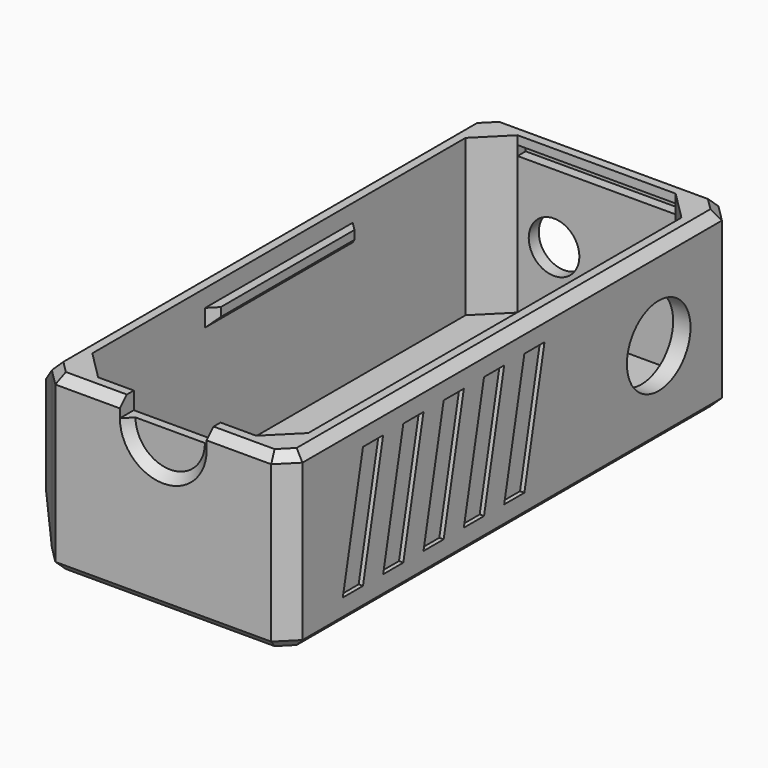
from build123d import *

# Parameters (mm, degrees)
F2_W      = 52
F2_H      = 116
F2_W_2    = 44.8
F2_H_2    = 108.8
F3_DEPTH  = 36
F4_DEPTH  = 3.6
F7_SIZE   = 3.6
F8_SIZE   = 5.9976
F6_R      = 5.25
F9_DEPTH  = 3.6
F5_R      = 8.25
F10_DEPTH = 3.6
F11_W     = 18
F11_H     = 3.6
F12_DEPTH = 3.6
F13_W     = 32.8048
F13_H     = 2
F14_DEPTH = 2.1
F6_R_2    = 12
F15_DEPTH = 1
F16_R     = 0.5
F17_W     = 38.28
F17_H     = 3.6
F19_DEPTH = 1.8
F18_W     = 38.28
F18_H     = 3.6
F20_DEPTH = 1.8
F21_SIZE  = 1.79999
F23_DEPTH = 1.8
F24_SIZE  = 1.79999
F26_W     = 89.2
F26_H     = 21.6
F27_DEPTH = 3.6
F28_DEPTH = 5.9976
F30_SIZE  = 3.59999
F29_W     = 4.775
F29_H     = 15.6718
F31_DEPTH = 2.9972
F32_SIZE  = 5.99759
F34_DEPTH = 0.9


# Not quite as in the source:
# - two fillets or chamfers of one size are made in one step
# - a fillet or chamfer is up to 0.001 mm smaller than in the source, because OpenCascade refuses the exact size


with BuildPart() as f3:
    # F2 (on Top) → F3 (new body)
    with BuildSketch(Plane.XY):
        Rectangle(F2_W, F2_H)
        Rectangle(F2_W_2, F2_H_2, mode=Mode.SUBTRACT)
    extrude(amount=F3_DEPTH)

    # F2 (on Top) → F4 (join)
    with BuildSketch(Plane.XY):
        Rectangle(F2_W_2, F2_H_2)
    extrude(amount=F4_DEPTH)

    # F7
    f7_edges = [f3.edges().sort_by_distance(p)[0] for p in [
        (-26, -58, 18),
        (26, -58, 18),
        (26, 58, 18),
        (-26, 58, 18),
    ]]
    chamfer(f7_edges, length=F7_SIZE)

    # F8
    f8_edges = [f3.edges().sort_by_distance(p)[0] for p in [
        (-22.4, 54.4, 19.8),
        (22.4, 54.4, 19.8),
        (-22.4, -54.4, 19.8),
        (22.4, -54.4, 19.8),
    ]]
    chamfer(f8_edges, length=F8_SIZE)

    # F6 (on face) → F9 (cut)
    with BuildSketch(Plane(origin=(0, 58, 0), x_dir=(-1, 0, 0), z_dir=(0, 1, 0))):
        with Locations((8.84, 18)):
            Circle(F6_R)
    extrude(amount=-F9_DEPTH, mode=Mode.SUBTRACT)

    # F5 (on face) → F10 (cut)
    with BuildSketch(Plane.YZ.offset(26)):
        with Locations((38, 18)):
            Circle(F5_R)
    extrude(amount=-F10_DEPTH, mode=Mode.SUBTRACT)

    # F11 (on face) → F12 (cut)
    with BuildSketch(Plane.XZ.offset(58)):
        with Locations((0, 34.2)):
            Rectangle(F11_W, F11_H)
    extrude(amount=-F12_DEPTH, mode=Mode.SUBTRACT)

    # F13 (on face) → F14 (cut)
    with BuildSketch(Plane.XZ.offset(-54.4)):
        with Locations((0, 33.2)):
            Rectangle(F13_W, F13_H)
    extrude(amount=-F14_DEPTH, mode=Mode.SUBTRACT)

    # F6 (on face) → F15 (cut)
    with BuildSketch(Plane(origin=(0, 58, 0), x_dir=(-1, 0, 0), z_dir=(0, 1, 0))):
        with Locations((8.84, 18)):
            Circle(F6_R_2)
        with Locations((8.84, 18)):
            Circle(F6_R, mode=Mode.SUBTRACT)
    extrude(amount=-F15_DEPTH, mode=Mode.SUBTRACT)

    # F16
    f16_edges = [f3.edges().sort_by_distance(p)[0] for p in [
        (0, 56.5, 34.2),
    ]]
    fillet(f16_edges, radius=F16_R)

    # F17 (on face) → F19 (join)
    with BuildSketch(Plane(origin=(22.4, 0, 0), x_dir=(0, -1, 0), z_dir=(-1, 0, 0))):
        with Locations((0, 30.6)):
            Rectangle(F17_W, F17_H)
    extrude(amount=F19_DEPTH)

    # F18 (on face) → F20 (join)
    with BuildSketch(Plane.YZ.offset(-22.4)):
        with Locations((0, 30.6)):
            Rectangle(F18_W, F18_H)
    extrude(amount=F20_DEPTH)

    # F21 (size 1.8 in the source; OpenCascade refuses exactly that, so slightly less here)
    f21_edges = [f3.edges().sort_by_distance(p)[0] for p in [
        (-20.6, -19.14, 30.6),
        (-20.6, 0, 28.8),
        (-20.6, 19.14, 30.6),
        (20.6, 19.14, 30.6),
        (20.6, 0, 28.8),
        (20.6, -19.14, 30.6),
        (-15.7, -58, 36),
        (-24.2, -56.2, 36),
        (-26, 0, 36),
        (-24.2, 56.2, 36),
        (0, 58, 36),
        (24.2, 56.2, 36),
        (26, 0, 36),
        (24.2, -56.2, 36),
        (15.7, -58, 36),
        (0, -58, 0),
        (-24.2, -56.2, 0),
        (-26, 0, 0),
        (-24.2, 56.2, 0),
        (0, 58, 0),
        (24.2, 56.2, 0),
        (26, 0, 0),
        (24.2, -56.2, 0),
    ]]
    chamfer(f21_edges, length=F21_SIZE)

    # F11 (on face) → F23 (cut)
    with BuildSketch(Plane.XZ.offset(58)):
        with BuildLine():
            ThreePointArc((-9, 32.4), (0, 23.4), (9, 32.4))
            Line((9, 32.4), (-9, 32.4))
        make_face()
    extrude(amount=-F23_DEPTH, mode=Mode.SUBTRACT)

    # F24 (size 1.8 in the source; OpenCascade refuses exactly that, so slightly less here)
    f24_edges = [f3.edges().sort_by_distance(p)[0] for p in [
        (0, -56.2, 23.4),
    ]]
    chamfer(f24_edges, length=F24_SIZE)

    # F26 (on face) → F27 (join)
    with BuildSketch(Plane(origin=(-26, 0, 0), x_dir=(0, -1, 0), z_dir=(-1, 0, 0))):
        with Locations((-9.8, 18)):
            Rectangle(F26_W, F26_H)
    extrude(amount=F27_DEPTH)

    # F26 (on face) → F28 (join)
    with BuildSketch(Plane(origin=(-26, 0, 0), x_dir=(0, -1, 0), z_dir=(-1, 0, 0))):
        Polygon((54.4, 1.8), (54.4, 34.2), (34.8, 34.2), (34.8, 28.8), (34.8, 7.2), (34.8, 1.8), align=None)
    extrude(amount=F28_DEPTH)

    # F30 (size 3.6 in the source; OpenCascade refuses exactly that, so slightly less here)
    f30_edges = [f3.edges().sort_by_distance(p)[0] for p in [
        (-29.6, 54.4, 18),
        (-29.6, 9.8, 7.2),
        (-29.6, 9.8, 28.8),
    ]]
    chamfer(f30_edges, length=F30_SIZE)

    # F29 (on face) → F31 (cut)
    with BuildSketch(Plane(origin=(-29.6, 0, 0), x_dir=(0, -1, 0), z_dir=(-1, 0, 0))):
        with Locations((-45.4, 18)):
            Rectangle(F29_W, F29_H)
        with Locations((-35.395, 18)):
            Rectangle(F29_W, F29_H)
        with Locations((-25.39, 18)):
            Rectangle(F29_W, F29_H)
        with Locations((-15.385, 18)):
            Rectangle(F29_W, F29_H)
        with Locations((-5.38, 18)):
            Rectangle(F29_W, F29_H)
        with Locations((4.625, 18)):
            Rectangle(F29_W, F29_H)
        with Locations((14.63, 18)):
            Rectangle(F29_W, F29_H)
        with Locations((24.635, 18)):
            Rectangle(F29_W, F29_H)
    extrude(amount=-F31_DEPTH, mode=Mode.SUBTRACT)

    # F32 (size 5.9976 in the source; OpenCascade refuses exactly that, so slightly less here)
    f32_edges = [f3.edges().sort_by_distance(p)[0] for p in [
        (-31.9976, -44.6, 34.2),
        (-31.9976, -54.4, 18),
        (-31.9976, -44.6, 1.8),
    ]]
    chamfer(f32_edges, length=F32_SIZE)

    # F33 (on face) → F34 (cut)
    with BuildSketch(Plane.YZ.offset(26)):
        Polygon((-33.4704, 30.7), (-38.7028, 30.7), (-43.9352, 5.3), (-38.7028, 5.3), align=None)
        Polygon((-23.0056, 30.7), (-28.238, 30.7), (-33.4704, 5.3), (-28.238, 5.3), align=None)
        Polygon((-12.5408, 30.7), (-17.7732, 30.7), (-23.0056, 5.3), (-17.7732, 5.3), align=None)
        Polygon((-2.076, 30.7), (-7.3084, 30.7), (-12.5408, 5.3), (-7.3084, 5.3), align=None)
        Polygon((8.3888, 30.7), (3.1564, 30.7), (-2.076, 5.3), (3.1564, 5.3), align=None)
    extrude(amount=-F34_DEPTH, mode=Mode.SUBTRACT)


solid = f3.part
